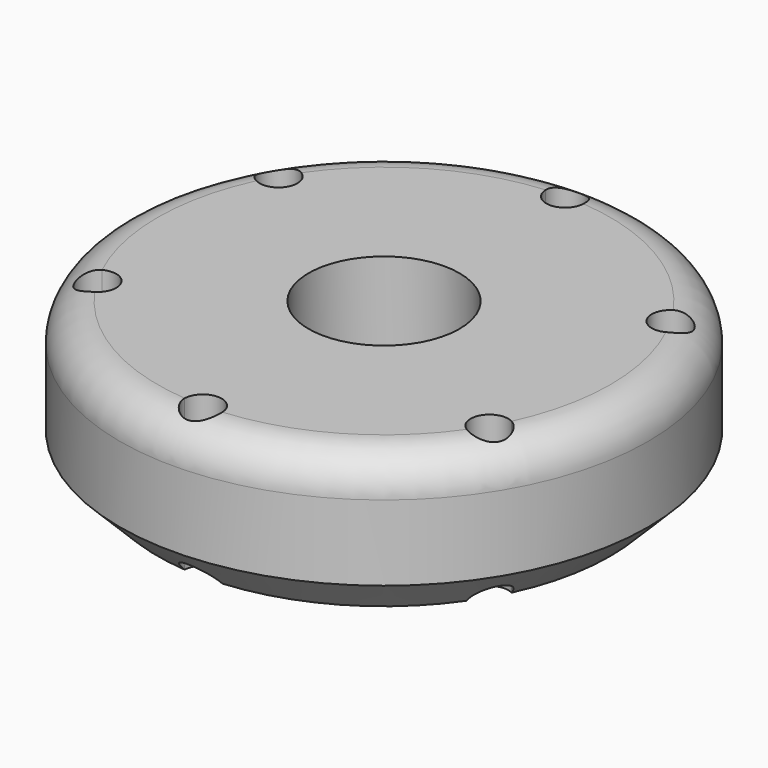
from build123d import *

# Parameters (mm, degrees)
F0_W     = 63.5
F0_H     = 50.8
F4_DEPTH = 76.201


# Not quite as in the source:
# - a fillet or chamfer that OpenCascade refuses, or shapes differently, is made with other operations: its cross-section is extruded or revolved along the edge and cut away or added


with BuildPart() as f1:
    # F0 (on Front) → F1 (revolve)
    with BuildSketch(Plane.XZ):
        with Locations((57.15, 25.4)):
            Rectangle(F0_W, F0_H)
    revolve(axis=Axis((0, 0, 63.5), (0, 0, 1)))

    # F3 (on offset) → F4 (cut, through all)
    with BuildSketch(Plane.XY.offset(76.2)):
        with BuildLine():
            ThreePointArc((0, 76.2), (3.175, 76.1338254326), (6.3444854527, 75.9354166667))
            ThreePointArc((6.3444854527, 75.9354166667), (6.3486212135, 76.0676796024), (6.35, 76.2))
            ThreePointArc((6.35, 76.2), (-0.1323203976, 82.5486212135), (-6.3444854527, 75.9354166667))
            ThreePointArc((-6.3444854527, 75.9354166667), (-3.175, 76.1338254326), (0, 76.2))
        make_face()
        with BuildLine():
            Line((0, 69.85), (0, 76.2))
            ThreePointArc((0, 76.2), (-3.175, 76.1338254326), (-6.3444854527, 75.9354166667))
            ThreePointArc((-6.3444854527, 75.9354166667), (-4.3955884608, 71.6172822383), (0, 69.85))
        make_face()
        with BuildLine():
            ThreePointArc((0, 69.85), (4.3955884608, 71.6172822383), (6.3444854527, 75.9354166667))
            ThreePointArc((6.3444854527, 75.9354166667), (3.175, 76.1338254326), (0, 76.2))
            Line((0, 76.2), (0, 69.85))
        make_face()
        with BuildLine():
            ThreePointArc((62.5897571539, 43.4621939093), (65.9911357684, 38.1), (68.9342426066, 32.4732227573))
            ThreePointArc((68.9342426066, 32.4732227573), (71.4230428194, 34.8110965675), (72.3411357684, 38.1))
            ThreePointArc((72.3411357684, 38.1), (69.0508535493, 43.6642274487), (62.5897571539, 43.4621939093))
        make_face()
        with BuildLine():
            ThreePointArc((62.5897571539, 43.4621939093), (60.4918744543, 34.925), (68.9342426066, 32.4732227573))
            ThreePointArc((68.9342426066, 32.4732227573), (65.9911357684, 38.1), (62.5897571539, 43.4621939093))
        make_face()
        with BuildLine():
            ThreePointArc((62.5897571539, -43.4621939093), (65.9911357684, -38.1), (68.9342426066, -32.4732227573))
            ThreePointArc((68.9342426066, -32.4732227573), (60.4918744543, -34.925), (62.5897571539, -43.4621939093))
        make_face()
        with BuildLine():
            ThreePointArc((72.3411357684, -38.1), (71.4230428194, -34.8110965675), (68.9342426066, -32.4732227573))
            ThreePointArc((68.9342426066, -32.4732227573), (65.9911357684, -38.1), (62.5897571539, -43.4621939093))
            ThreePointArc((62.5897571539, -43.4621939093), (69.0508535493, -43.6642274487), (72.3411357684, -38.1))
        make_face()
        with BuildLine():
            ThreePointArc((-6.3444854527, -75.9354166667), (0, -76.2), (6.3444854527, -75.9354166667))
            ThreePointArc((6.3444854527, -75.9354166667), (0, -69.85), (-6.3444854527, -75.9354166667))
        make_face()
        with BuildLine():
            ThreePointArc((6.35, -76.2), (6.3486212135, -76.0676796024), (6.3444854527, -75.9354166667))
            ThreePointArc((6.3444854527, -75.9354166667), (0, -76.2), (-6.3444854527, -75.9354166667))
            ThreePointArc((-6.3444854527, -75.9354166667), (-0.1323203976, -82.5486212135), (6.35, -76.2))
        make_face()
        with BuildLine():
            ThreePointArc((-68.9342426066, -32.4732227573), (-71.4903970824, -41.275), (-62.5897571539, -43.4621939093))
            ThreePointArc((-62.5897571539, -43.4621939093), (-65.9911357684, -38.1), (-68.9342426066, -32.4732227573))
        make_face()
        with BuildLine():
            ThreePointArc((-68.9342426066, -32.4732227573), (-65.9911357684, -38.1), (-62.5897571539, -43.4621939093))
            ThreePointArc((-62.5897571539, -43.4621939093), (-60.4269083197, -41.159717781), (-59.6411357684, -38.1))
            ThreePointArc((-59.6411357684, -38.1), (-62.7022323358, -32.6680929489), (-68.9342426066, -32.4732227573))
        make_face()
        with BuildLine():
            ThreePointArc((-68.9342426066, 32.4732227573), (-65.9911357684, 38.1), (-62.5897571539, 43.4621939093))
            ThreePointArc((-62.5897571539, 43.4621939093), (-71.4903970824, 41.275), (-68.9342426066, 32.4732227573))
        make_face()
        with BuildLine():
            ThreePointArc((-59.6411357684, 38.1), (-60.4269083197, 41.159717781), (-62.5897571539, 43.4621939093))
            ThreePointArc((-62.5897571539, 43.4621939093), (-65.9911357684, 38.1), (-68.9342426066, 32.4732227573))
            ThreePointArc((-68.9342426066, 32.4732227573), (-62.7022323358, 32.6680929489), (-59.6411357684, 38.1))
        make_face()
    extrude(amount=-F4_DEPTH, mode=Mode.SUBTRACT)

    # F5: fillet of radius 12.7 on 1 edges, made by hand

    # F5_s1 → F5_t2 (revolve, cut)
    with BuildSketch(Plane.XZ):
        with BuildLine():
            ThreePointArc((76.2, 50.8), (85.1802561211, 47.0802561211), (88.9, 38.1))
            Line((88.9, 38.1), (88.9, 50.8))
            Line((88.9, 50.8), (76.2, 50.8))
        make_face()
    revolve(axis=Axis((0, 0, 50.8), (0, 0, 1)), mode=Mode.SUBTRACT)

    # F6: chamfer of 12.7 on 3 edges, made by hand

    # F6_s1 → F6_t2 (revolve, cut)
    with BuildSketch(Plane.XZ):
        Polygon((76.2, 0), (88.9, 12.7), (88.9, 0), align=None)
    revolve(axis=Axis((0, 0, 0), (0, 0, 1)), mode=Mode.SUBTRACT)


solid = f1.part
